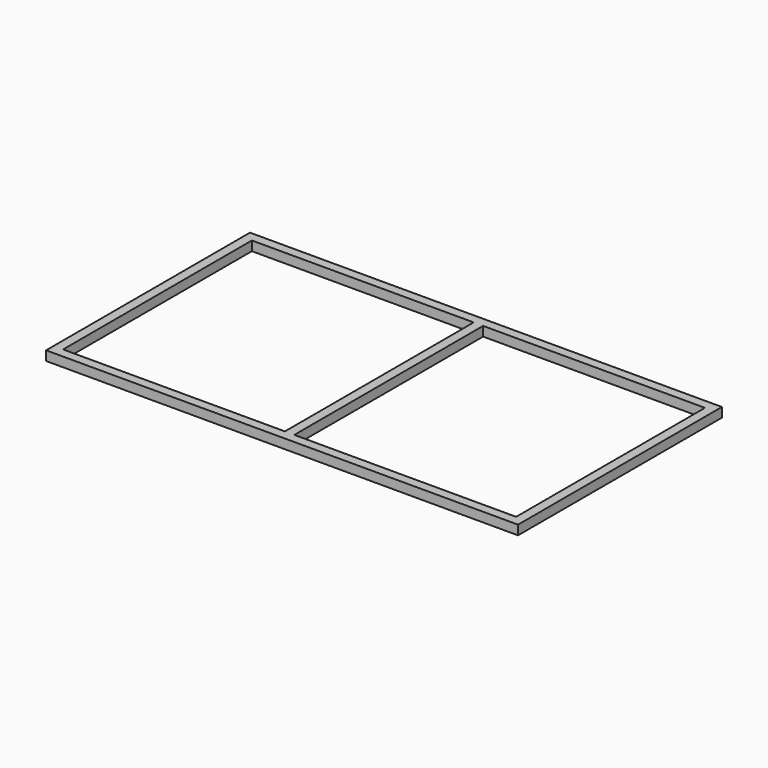
from build123d import *

# Parameters (mm, degrees)
F0_W     = 40
F0_H     = 40
F0_H_2   = 1000
F1_DEPTH = 3
F2_W     = 2000
F2_H     = 1080
F2_W_2   = 1994
F2_H_2   = 1074
F2_W_3   = 1926
F2_H_3   = 1006
F2_W_4   = 40
F2_H_4   = 1000
F2_W_5   = 34
F2_H_5   = 994
F3_DEPTH = 34
F4_W     = 2000
F4_H     = 1080
F4_W_2   = 40
F4_H_2   = 1000
F4_W_3   = 34
F4_H_3   = 994
F5_DEPTH = 3


with BuildPart() as f1:
    # F0 (on Top) → F1 (new body)
    with BuildSketch(Plane.XY):
        with Locations((0, 520)):
            Rectangle(F0_W, F0_H)
        Polygon((-20, 500), (-20, 540), (-1000, 540), (-1000, -540), (-20, -540), (-20, -500), (-960, -500), (-960, 500), align=None)
        Polygon((1000, 540), (20, 540), (20, 500), (960, 500), (960, -500), (20, -500), (20, -540), (1000, -540), align=None)
        with Locations((0, -520)):
            Rectangle(F0_W, F0_H)
        Rectangle(F0_W, F0_H_2)
    extrude(amount=F1_DEPTH)

    # F2 (on face) → F3 (join)
    with BuildSketch(Plane.XY.offset(3)):
        Rectangle(F2_W, F2_H)
        Rectangle(F2_W_2, F2_H_2, mode=Mode.SUBTRACT)
        Rectangle(F2_W_3, F2_H_3)
        Polygon((-20, 500), (20, 500), (960, 500), (960, -500), (20, -500), (-20, -500), (-960, -500), (-960, 500), align=None, mode=Mode.SUBTRACT)
        Rectangle(F2_W_4, F2_H_4)
        Rectangle(F2_W_5, F2_H_5, mode=Mode.SUBTRACT)
    extrude(amount=F3_DEPTH)

    # F4 (on face) → F5 (join)
    with BuildSketch(Plane.XY.offset(37)):
        Rectangle(F4_W, F4_H)
        Polygon((20, 500), (960, 500), (960, -500), (20, -500), (-20, -500), (-960, -500), (-960, 500), (-20, 500), align=None, mode=Mode.SUBTRACT)
        Rectangle(F4_W_2, F4_H_2)
        Rectangle(F4_W_3, F4_H_3, mode=Mode.SUBTRACT)
        Rectangle(F4_W_3, F4_H_3)
    extrude(amount=F5_DEPTH)


solid = f1.part
